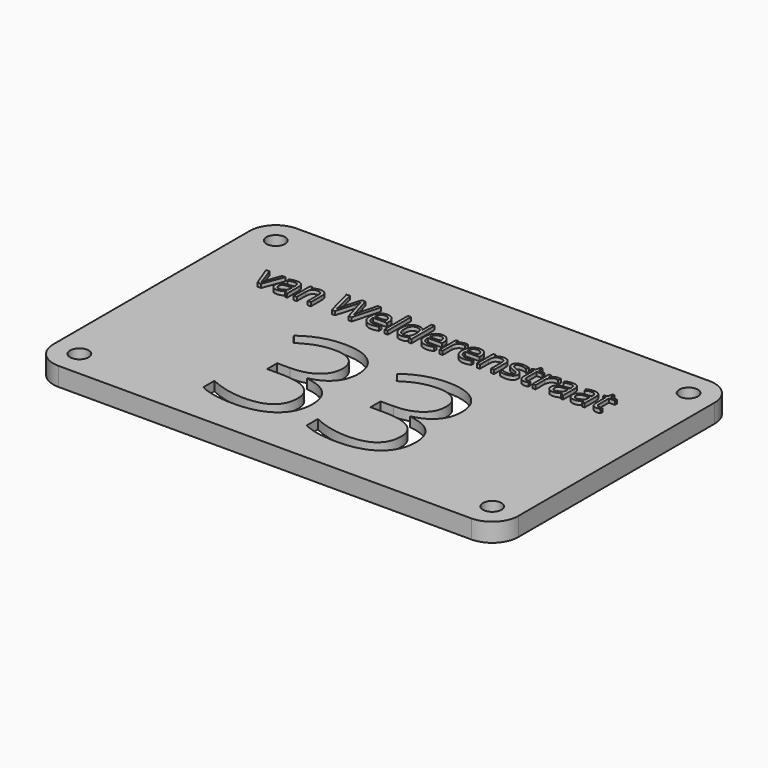
from build123d import *

# Parameters (mm, degrees)
F0_R         = 2.5
F1_DEPTH     = 5
F3_DEPTH     = 2.5
F4_TEXT_SIZE = 10.3543997684
F5_DEPTH     = 1
F6_TEXT_SIZE = 48.6111111111
F7_DEPTH     = 6.0010001


# Not quite as in the source:
# - Text() gives the source's letters only with a copy of the font that has no kerning and outlines rounded to 1/6400 em; it was checked with that copy


with BuildPart() as f1:
    # F0 (on Top) → F1 (new body)
    with BuildSketch(Plane.XY):
        with BuildLine():
            Line((-55.5, -40), (55.5, -40))
            ThreePointArc((55.5, -40), (60.4497474683, -37.9497474683), (62.5, -33))
            Line((62.5, -33), (62.5, 33))
            ThreePointArc((62.5, 33), (60.4497474683, 37.9497474683), (55.5, 40))
            Line((55.5, 40), (-55.5, 40))
            ThreePointArc((-55.5, 40), (-60.4497474683, 37.9497474683), (-62.5, 33))
            Line((-62.5, 33), (-62.5, -33))
            ThreePointArc((-62.5, -33), (-60.4497474683, -37.9497474683), (-55.5, -40))
        make_face()
        with Locations((-55.5, -33)):
            Circle(F0_R, mode=Mode.SUBTRACT)
        with Locations((55.5, -33)):
            Circle(F0_R, mode=Mode.SUBTRACT)
        with Locations((-55.5, 33)):
            Circle(F0_R, mode=Mode.SUBTRACT)
        with Locations((55.5, 33)):
            Circle(F0_R, mode=Mode.SUBTRACT)
    extrude(amount=F1_DEPTH)

    # F2 (on Top) → F3 (cut)
    with BuildSketch(Plane.XY):
        with BuildLine():
            ThreePointArc((52.5, 28), (51.9142135624, 29.4142135624), (50.5, 30))
            Line((50.5, 30), (-50.5, 30))
            ThreePointArc((-50.5, 30), (-51.9142135624, 29.4142135624), (-52.5, 28))
            Line((-52.5, 28), (-52.5, -28))
            ThreePointArc((-52.5, -28), (-51.9142135624, -29.4142135624), (-50.5, -30))
            Line((-50.5, -30), (50.5, -30))
            ThreePointArc((50.5, -30), (51.9142135624, -29.4142135624), (52.5, -28))
            Line((52.5, -28), (52.5, 28))
        make_face()
    extrude(amount=F3_DEPTH, mode=Mode.SUBTRACT)

    # F4 (on face) → F5 (join)
    with BuildSketch(Plane.XY.offset(5)):
        with Locations((-47.5, 14.210501422)):
            Text('van Welderenstraat', F4_TEXT_SIZE, font='Open Sans', text_align=(TextAlign.LEFT, TextAlign.BOTTOM))
    extrude(amount=F5_DEPTH)

    # F6 (on Top) → F7 (cut, through all)
    with BuildSketch(Plane.XY):
        with Locations((-27.9437934028, -30)):
            Text('33', F6_TEXT_SIZE, font='Open Sans', text_align=(TextAlign.LEFT, TextAlign.BOTTOM))
    extrude(amount=F7_DEPTH, mode=Mode.SUBTRACT)


solid = f1.part
